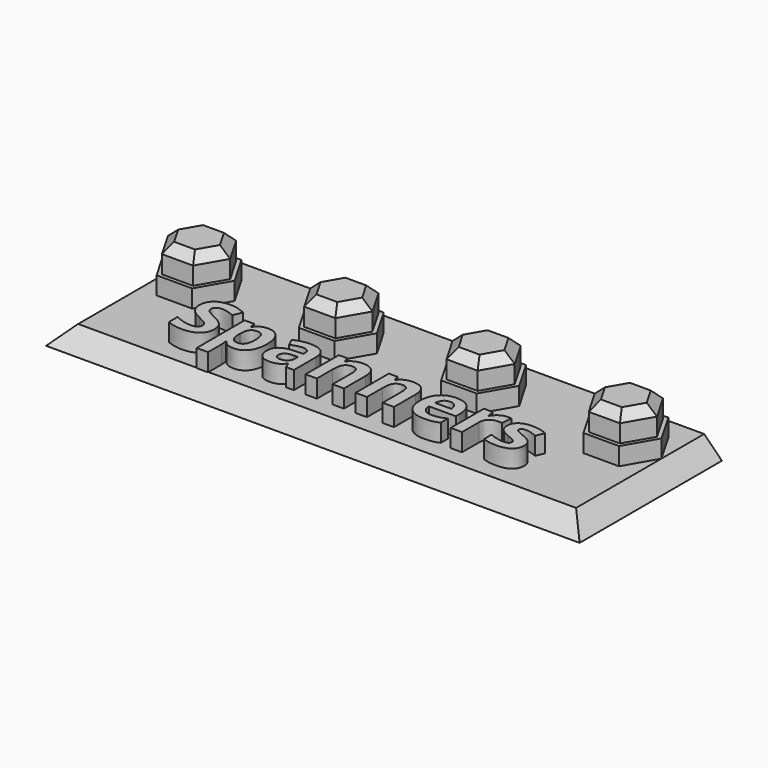
from build123d import *

# Parameters (mm, degrees)
F0_W          = 76.2
F0_H          = 25.4
F1_DEPTH      = 2.54
F3_DEPTH      = 2.54
F3_DEPTH_BACK = 2.54
F5_DEPTH      = 3.81
F6_SIZE       = 1.27
F7_SIZE       = 2.53999
F8_TEXT_SIZE  = 10.8761248453
F9_DEPTH      = 2.54


# Not quite as in the source:
# - a fillet or chamfer is up to 0.001 mm smaller than in the source, because OpenCascade refuses the exact size
# - Text() gives the source's letters only with a copy of the font that has no kerning and outlines rounded to 1/6400 em; it was checked with that copy


with BuildPart() as f1:
    # F0 (on Top) → F1 (new body)
    with BuildSketch(Plane.XY):
        with Locations((-14.717983855, 80.0740443289)):
            Rectangle(F0_W, F0_H)
        Polygon((-42.657983855, 89.5534533801), (-40.117983855, 85.1540443289), (-42.657983855, 80.7546352776), (-47.737983855, 80.7546352776), (-50.277983855, 85.1540443289), (-47.737983855, 89.5534533801), align=None, mode=Mode.SUBTRACT)
        Polygon((-27.417983855, 89.5534533801), (-22.337983855, 89.5534533801), (-19.797983855, 85.1540443289), (-22.337983855, 80.7546352776), (-27.417983855, 80.7546352776), (-29.957983855, 85.1540443289), align=None, mode=Mode.SUBTRACT)
        Polygon((-7.097983855, 89.5534533801), (-2.017983855, 89.5534533801), (0.522016145, 85.1540443289), (-2.017983855, 80.7546352776), (-7.097983855, 80.7546352776), (-9.637983855, 85.1540443289), align=None, mode=Mode.SUBTRACT)
        Polygon((13.222016145, 89.5534533801), (18.302016145, 89.5534533801), (20.842016145, 85.1540443289), (18.302016145, 80.7546352776), (13.222016145, 80.7546352776), (10.682016145, 85.1540443289), align=None, mode=Mode.SUBTRACT)
    extrude(amount=F1_DEPTH)

    # F2 (on face) → F3 (join, two sides)
    with BuildSketch(Plane.XY.offset(2.54)) as f3_sk:
        Polygon((-42.657983855, 89.5534533801), (-47.737983855, 89.5534533801), (-50.277983855, 85.1540443289), (-47.737983855, 80.7546352776), (-42.657983855, 80.7546352776), (-40.117983855, 85.1540443289), align=None)
        Polygon((-22.337983855, 89.5534533801), (-27.417983855, 89.5534533801), (-29.957983855, 85.1540443289), (-27.417983855, 80.7546352776), (-22.337983855, 80.7546352776), (-19.797983855, 85.1540443289), align=None)
        Polygon((-7.097983855, 89.5534533801), (-9.637983855, 85.1540443289), (-7.097983855, 80.7546352776), (-2.017983855, 80.7546352776), (0.522016145, 85.1540443289), (-2.017983855, 89.5534533801), align=None)
        Polygon((20.842016145, 85.1540443289), (18.302016145, 89.5534533801), (13.222016145, 89.5534533801), (10.682016145, 85.1540443289), (13.222016145, 80.7546352776), (18.302016145, 80.7546352776), align=None)
    extrude(amount=F3_DEPTH)
    extrude(f3_sk.sketch, amount=-F3_DEPTH_BACK)

    # F4 (on face) → F5 (join)
    with BuildSketch(Plane.XY.offset(5.08)):
        Polygon((-42.975483855, 89.0035272487), (-45.197983855, 89.0035272487), (-45.197983855, 81.304561409), (-42.975483855, 81.304561409), (-40.752983855, 85.1540443289), align=None)
        Polygon((-45.197983855, 81.304561409), (-45.197983855, 89.0035272487), (-47.420483855, 89.0035272487), (-49.642983855, 85.1540443289), (-47.420483855, 81.304561409), align=None)
        Polygon((-22.655483855, 81.304561409), (-20.432983855, 85.1540443289), (-22.655483855, 89.0035272487), (-27.100483855, 89.0035272487), (-29.322983855, 85.1540443289), (-27.100483855, 81.304561409), align=None)
        Polygon((-2.335483855, 81.304561409), (-0.112983855, 85.1540443289), (-2.335483855, 89.0035272487), (-6.780483855, 89.0035272487), (-9.002983855, 85.1540443289), (-6.780483855, 81.304561409), align=None)
        Polygon((17.984516145, 81.304561409), (20.207016145, 85.1540443289), (17.984516145, 89.0035272487), (13.539516145, 89.0035272487), (11.317016145, 85.1540443289), (13.539516145, 81.304561409), align=None)
    extrude(amount=F5_DEPTH)

    # F6
    f6_edges = [f1.edges().sort_by_distance(p)[0] for p in [
        (-45.197984, 81.304561, 8.89),
        (-41.864234, 83.229303, 8.89),
        (-45.197984, 89.003527, 8.89),
        (-48.531734, 87.078786, 8.89),
        (-48.531734, 83.229303, 8.89),
        (-41.864234, 87.078786, 8.89),
        (-28.211734, 87.078786, 8.89),
        (-24.877984, 89.003527, 8.89),
        (-21.544234, 87.078786, 8.89),
        (-21.544234, 83.229303, 8.89),
        (-24.877984, 81.304561, 8.89),
        (-28.211734, 83.229303, 8.89),
        (-4.557984, 81.304561, 8.89),
        (-1.224234, 83.229303, 8.89),
        (-1.224234, 87.078786, 8.89),
        (-4.557984, 89.003527, 8.89),
        (-7.891734, 87.078786, 8.89),
        (-7.891734, 83.229303, 8.89),
        (15.762016, 81.304561, 8.89),
        (12.428266, 83.229303, 8.89),
        (12.428266, 87.078786, 8.89),
        (15.762016, 89.003527, 8.89),
        (19.095766, 87.078786, 8.89),
        (19.095766, 83.229303, 8.89),
    ]]
    chamfer(f6_edges, length=F6_SIZE)

    # F7 (size 2.54 in the source; OpenCascade refuses exactly that, so slightly less here)
    f7_edges = [f1.edges().sort_by_distance(p)[0] for p in [
        (-52.817984, 80.074044, 2.54),
        (-14.717984, 67.374044, 2.54),
        (23.382016, 80.074044, 2.54),
    ]]
    chamfer(f7_edges, length=F7_SIZE)

    # F8 (on face) → F9 (join)
    with BuildSketch(Plane.XY.offset(2.54)):
        with Locations((-40.117983855, 72.4540443289)):
            Text('Spanners', F8_TEXT_SIZE, font='Open Sans', font_style=FontStyle.BOLD, text_align=(TextAlign.LEFT, TextAlign.BOTTOM))
    extrude(amount=F9_DEPTH)


solid = f1.part
